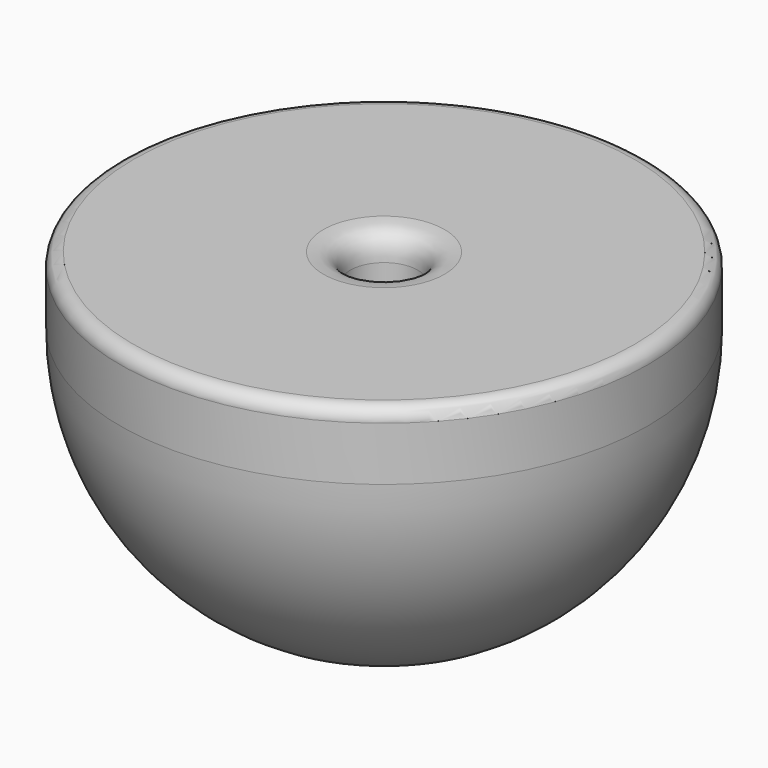
from build123d import *

# Parameters (mm, degrees)
F2_R     = 49.784
F2_R_2   = 6.35
F3_DEPTH = 12.7
F4_R     = 2.54
F6_DEPTH = 15.24
F7_R     = 1.27


# Not quite as in the source:
# - a fillet or chamfer that OpenCascade refuses, or shapes differently, is made with other operations: its cross-section is extruded or revolved along the edge and cut away or added


with BuildPart() as f1:
    # F0 (on Front) → F1 (revolve)
    with BuildSketch(Plane.XZ):
        with BuildLine():
            Line((0, 0), (-49.784, 0))
            ThreePointArc((-49.784, 0), (-35.2026039946, -35.2026039946), (0, -49.784))
            Line((0, -49.784), (0, 0))
        make_face()
    revolve(axis=Axis((0, 0, -24.892), (0, 0, -1)))

    # F2 (on face) → F3 (join)
    with BuildSketch(Plane.XY):
        Circle(F2_R)
        Circle(F2_R_2, mode=Mode.SUBTRACT)
    extrude(amount=F3_DEPTH)

    # F4
    f4_edges = [f1.edges().sort_by_distance(p)[0] for p in [
        (-49.784, 0, 12.7),
    ]]
    fillet(f4_edges, radius=F4_R)

    # F5: fillet of radius 5.08 on 1 edges, made by hand

    # F5_s1 → F5_t2 (revolve, cut)
    with BuildSketch(Plane.XZ):
        with BuildLine():
            add(Edge.make_bspline(
                [(11.43, 12.7), (6.35, 12.7), (6.35, 7.62)],
                knots=[0, 0, 0, 1, 1, 1], degree=2, weights=[1, 1, 1]))
            Line((6.35, 7.62), (6.35, 12.7))
            Line((6.35, 12.7), (11.43, 12.7))
        make_face()
    revolve(axis=Axis((0, 0, 12.7), (0, 0, 1)), mode=Mode.SUBTRACT)

    # F6 (cut): a face of the model
    f6_faces = [f1.faces().sort_by_distance(p)[0] for p in [
        (0, 0, 0),
    ]]
    extrude(f6_faces, amount=-F6_DEPTH, mode=Mode.SUBTRACT)

    # F7
    f7_edges = [f1.edges().sort_by_distance(p)[0] for p in [
        (-6.35, 0, -15.24),
    ]]
    fillet(f7_edges, radius=F7_R)


solid = f1.part
